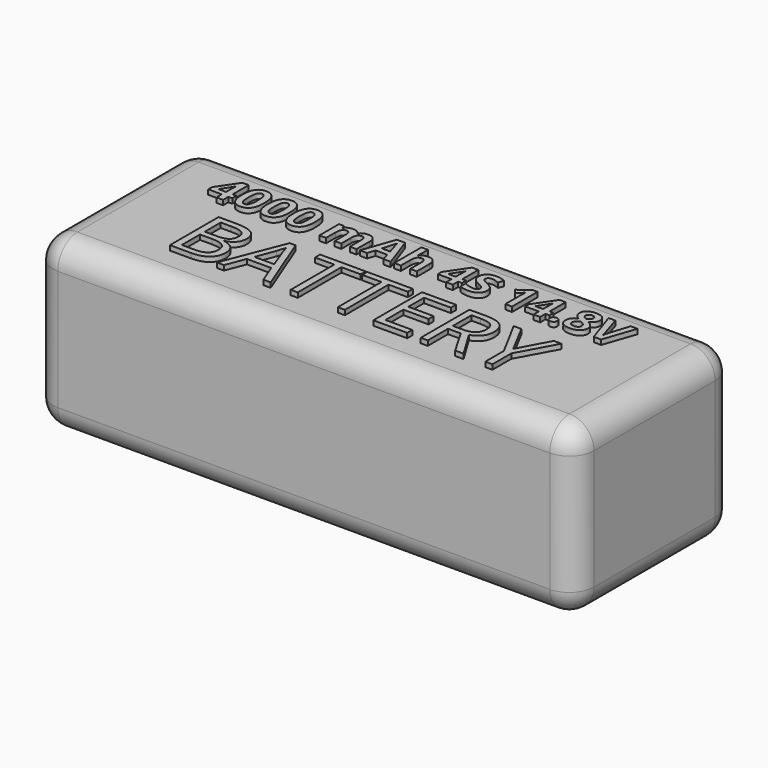
from build123d import *

# Parameters (mm, degrees)
F0_W           = 112
F0_H           = 35
F1_DEPTH       = 41.5
F3_DEPTH       = 1
F4_R           = 5.08
F5_TEXT_SIZE   = 9.2628987558
F5_TEXT_SIZE_2 = 17.6388888889
F6_DEPTH       = 1
F7_TEXT_SIZE   = 20.8333333333
F8_DEPTH       = 1
F9_TEXT_SIZE   = 20.8333333333
F10_DEPTH      = 1


# Not quite as in the source:
# - Text() gives the source's letters only with a copy of the font that has no kerning and outlines rounded to 1/6400 em; it was checked with that copy


with BuildPart() as f1:
    # F0 (on Front) → F1 (new body)
    with BuildSketch(Plane.XZ):
        with Locations((56, -17.5)):
            Rectangle(F0_W, F0_H)
    extrude(amount=F1_DEPTH)

    # F4
    f4_edges = [f1.edges().sort_by_distance(p)[0] for p in [
        (112, -20.75, 0),
        (0, -20.75, 0),
        (56, 0, 0),
        (56, -41.5, 0),
        (112, -20.75, -35),
        (112, 0, -17.5),
        (112, -41.5, -17.5),
        (0, -41.5, -17.5),
        (56, -41.5, -35),
        (0, 0, -17.5),
        (56, 0, -35),
        (0, -20.75, -35),
    ]]
    fillet(f4_edges, radius=F4_R)


with BuildPart() as f3:
    # F2 (on face) → F3 (new body)
    with BuildSketch(Plane(origin=(0, 0, -35), x_dir=(1, 0, 0), z_dir=(0, 0, -1))):
        Polygon((43.6396710575, 33.25), (13.5, 33.25), (13.5, 17.7942663431), (13.5, 8.25), (68.9369663596, 8.25), (98.5, 8.25), (98.5, 17.5642911345), (98.5, 33.25), align=None)
    extrude(amount=F3_DEPTH)

    # F7 (on face) → F8 (cut)
    with BuildSketch(Plane(origin=(0, 0, -36), x_dir=(1, 0, 0), z_dir=(0, 0, -1))):
        with Locations((15.6370442708, 13.25)):
            Text('VELCRO', F7_TEXT_SIZE, font='Open Sans', font_style=FontStyle.BOLD, text_align=(TextAlign.LEFT, TextAlign.BOTTOM))
    extrude(amount=-F8_DEPTH, mode=Mode.SUBTRACT)


with BuildPart() as f6:
    # F5 (on face) → F6 (new body)
    with BuildSketch(Plane.XY):
        with Locations((13.2727084971, -14.400921762)):
            Text('4000 mAh 4S 14.8V', F5_TEXT_SIZE, font='Open Sans', font_style=FontStyle.BOLD, text_align=(TextAlign.LEFT, TextAlign.BOTTOM))
        with Locations((19.0782226562, -32.1603800774)):
            Text('BATTERY', F5_TEXT_SIZE_2, font='Open Sans', text_align=(TextAlign.LEFT, TextAlign.BOTTOM))
    extrude(amount=F6_DEPTH)


with BuildPart() as f10:
    # F9 (on face) → F10 (new body)
    with BuildSketch(Plane(origin=(0, 0, -35), x_dir=(1, 0, 0), z_dir=(0, 0, -1))):
        with Locations((15.6370442708, 13.25)):
            Text('VELCRO', F9_TEXT_SIZE, font='Open Sans', font_style=FontStyle.BOLD, text_align=(TextAlign.LEFT, TextAlign.BOTTOM))
    extrude(amount=F10_DEPTH)


solid = Compound([f1.part, f3.part, f6.part, f10.part])
